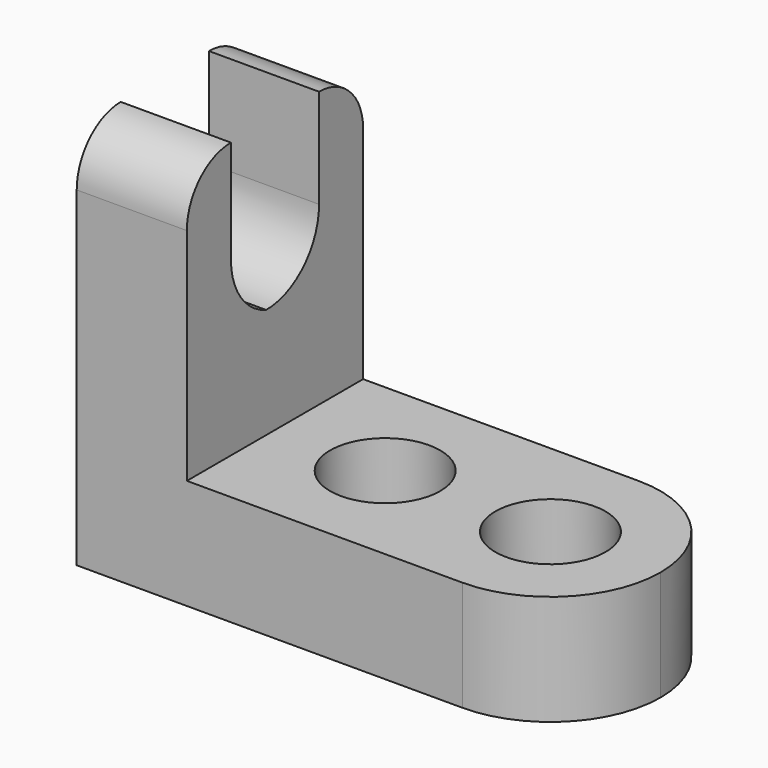
from build123d import *

# Parameters (mm, degrees)
F1_DEPTH     = 25.4
F2_R         = 12.7
F3_R         = 12.69999
F4_R         = 6.35
F5_DEPTH     = 25.4
F6_R         = 6.35
F7_R         = 6.35
F8_W         = 12.7
F8_H         = 19.05
F9_DEPTH     = 25.4
F10_R        = 7.62
F11_T1_DEPTH = 12.7


# Not quite as in the source:
# - a fillet or chamfer that OpenCascade refuses, or shapes differently, is made with other operations: its cross-section is extruded or revolved along the edge and cut away or added
# - a fillet or chamfer is up to 0.001 mm smaller than in the source, because OpenCascade refuses the exact size


with BuildPart() as f1:
    # F0 (on Front) → F1 (new body)
    with BuildSketch(Plane.XZ):
        Polygon((0, 0), (57.15, 0), (57.15, 12.7), (12.7, 12.7), (12.7, 44.45), (0, 44.45), align=None)
    extrude(amount=F1_DEPTH)

    # F2
    f2_edges = [f1.edges().sort_by_distance(p)[0] for p in [
        (57.15, -25.4, 6.35),
    ]]
    fillet(f2_edges, radius=F2_R)

    # F3 (radius 12.7 in the source; OpenCascade refuses exactly that, so slightly less here)
    f3_edges = [f1.edges().sort_by_distance(p)[0] for p in [
        (57.15, 0, 6.35),
    ]]
    fillet(f3_edges, radius=F3_R)

    # F4 (on face) → F5 (cut)
    with BuildSketch(Plane.XY.offset(12.7)):
        with Locations((44.45, -12.7)):
            Circle(F4_R)
        with Locations((25.4, -12.7)):
            Circle(F4_R)
    extrude(amount=-F5_DEPTH, mode=Mode.SUBTRACT)

    # F6
    f6_edges = [f1.edges().sort_by_distance(p)[0] for p in [
        (6.35, -25.4, 44.45),
    ]]
    fillet(f6_edges, radius=F6_R)

    # F7
    f7_edges = [f1.edges().sort_by_distance(p)[0] for p in [
        (6.35, 0, 44.45),
    ]]
    fillet(f7_edges, radius=F7_R)

    # F8 (on face) → F9 (cut)
    with BuildSketch(Plane.YZ.offset(12.7)):
        with Locations((-12.7, 34.925)):
            Rectangle(F8_W, F8_H)
    extrude(amount=-F9_DEPTH, mode=Mode.SUBTRACT)

    # F10
    f10_edges = [f1.edges().sort_by_distance(p)[0] for p in [
        (6.35, -6.35, 25.4),
    ]]
    fillet(f10_edges, radius=F10_R)

    # F11: fillet of radius 7.62 on 1 edges, made by hand

    # F11_s2 → F11_t1 (join)
    with BuildSketch(Plane.YZ):
        with BuildLine():
            ThreePointArc((-13.97, 25.4), (-17.6517039467, 28.1847958456), (-19.05, 32.5842048969))
            Line((-19.05, 32.5842048969), (-19.05, 25.4))
            Line((-19.05, 25.4), (-13.97, 25.4))
        make_face()
    extrude(amount=F11_T1_DEPTH)


solid = f1.part
